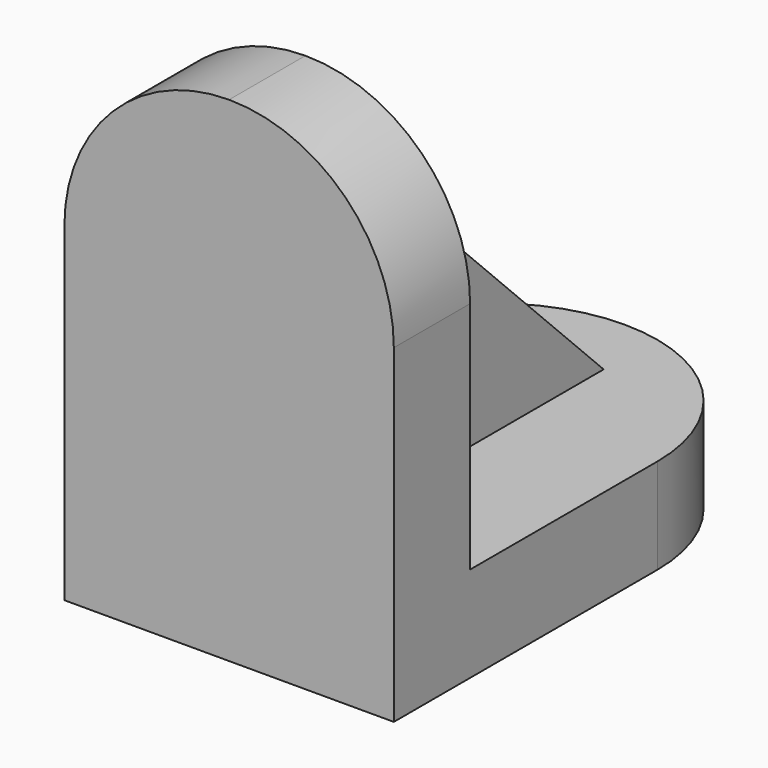
from build123d import *

# Parameters (mm, degrees)
F1_DEPTH = 38
F2_R     = 18.99999
F3_R     = 18.99999
F6_DEPTH = 8


# Not quite as in the source:
# - a fillet or chamfer is up to 0.001 mm smaller than in the source, because OpenCascade refuses the exact size


with BuildPart() as f1:
    # F0 (on Right) → F1 (new body)
    with BuildSketch(Plane.YZ):
        Polygon((-14.4942225739, 53.3158381923), (-14.4942225739, -3.6841618077), (42.5057774261, -3.6841618077), (42.5057774261, 7.3158381923), (-3.4942225739, 7.3158381923), (-3.4942225739, 53.3158381923), align=None)
    extrude(amount=F1_DEPTH)

    # F2 (radius 19 in the source; OpenCascade refuses exactly that, so slightly less here)
    f2_edges = [f1.edges().sort_by_distance(p)[0] for p in [
        (38, -8.994223, 53.315838),
        (0, -8.994223, 53.315838),
    ]]
    fillet(f2_edges, radius=F2_R)

    # F3 (radius 19 in the source; OpenCascade refuses exactly that, so slightly less here)
    f3_edges = [f1.edges().sort_by_distance(p)[0] for p in [
        (38, 42.505777, 1.815838),
        (0, 42.505777, 1.815838),
    ]]
    fillet(f3_edges, radius=F3_R)

    # F5 (on offset) → F6 (join)
    with BuildSketch(Plane.YZ.offset(15)):
        Polygon((34.5057774261, 7.3158381923), (-3.4942225739, 45.3158381923), (-3.4942225739, 7.3158381923), align=None)
    extrude(amount=F6_DEPTH)


solid = f1.part
